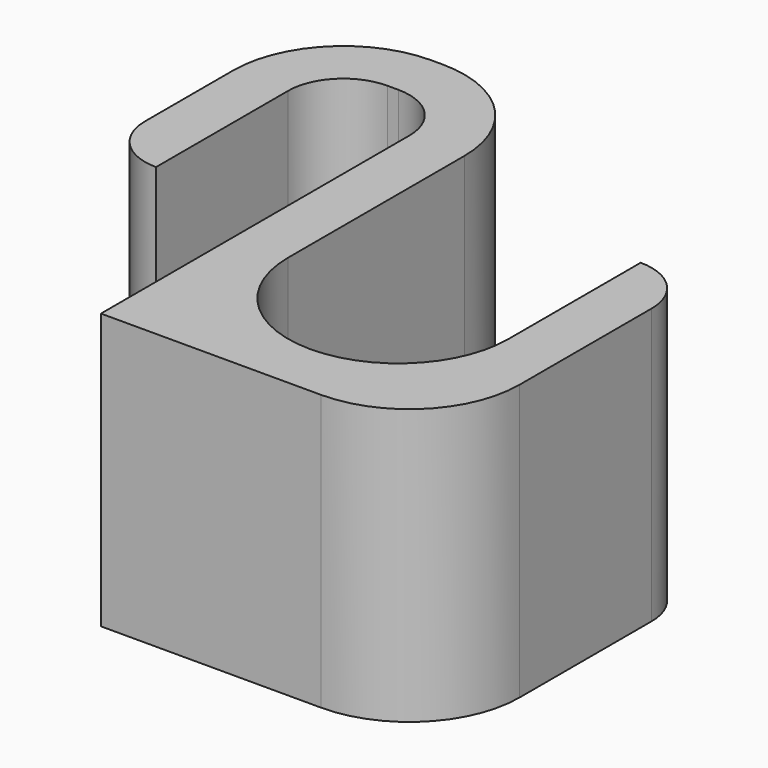
from build123d import *

# Parameters (mm, degrees)
F1_DEPTH = 25
F2_R     = 4.99999
F3_R     = 4.99999


# Not quite as in the source:
# - a fillet or chamfer is up to 0.001 mm smaller than in the source, because OpenCascade refuses the exact size


with BuildPart() as f1:
    # F0 (on Top) → F1 (new body)
    with BuildSketch(Plane.XY):
        with BuildLine():
            Line((-16, 0), (-11, 0))
            Line((-11, 0), (-11, 15))
            ThreePointArc((-11, 15), (-9.5355339059, 18.5355339059), (-6, 20))
            Line((-6, 20), (-5, 20))
            ThreePointArc((-5, 20), (-1.4644660941, 18.5355339059), (0, 15))
            Line((0, 15), (0, -20))
            Line((0, -20), (20, -20))
            ThreePointArc((20, -20), (27.0710678119, -17.0710678119), (30, -10))
            Line((30, -10), (30, 10))
            Line((30, 10), (25, 10))
            Line((25, 10), (25, -1.100000754))
            Line((25, -1.100000754), (25, -5))
            ThreePointArc((25, -5), (22.0710678119, -12.0710678119), (15, -15))
            ThreePointArc((15, -15), (7.9289321881, -12.0710678119), (5, -5))
            Line((5, -5), (5, 15))
            ThreePointArc((5, 15), (2.0710678119, 22.0710678119), (-5, 25))
            Line((-5, 25), (-6, 25))
            ThreePointArc((-6, 25), (-13.0710678119, 22.0710678119), (-16, 15))
            Line((-16, 15), (-16, 0))
        make_face()
    extrude(amount=F1_DEPTH)

    # F2 (radius 5 in the source; OpenCascade refuses exactly that, so slightly less here)
    f2_edges = [f1.edges().sort_by_distance(p)[0] for p in [
        (30, 10, 12.5),
    ]]
    fillet(f2_edges, radius=F2_R)

    # F3 (radius 5 in the source; OpenCascade refuses exactly that, so slightly less here)
    f3_edges = [f1.edges().sort_by_distance(p)[0] for p in [
        (-16, 0, 12.5),
    ]]
    fillet(f3_edges, radius=F3_R)


solid = f1.part
